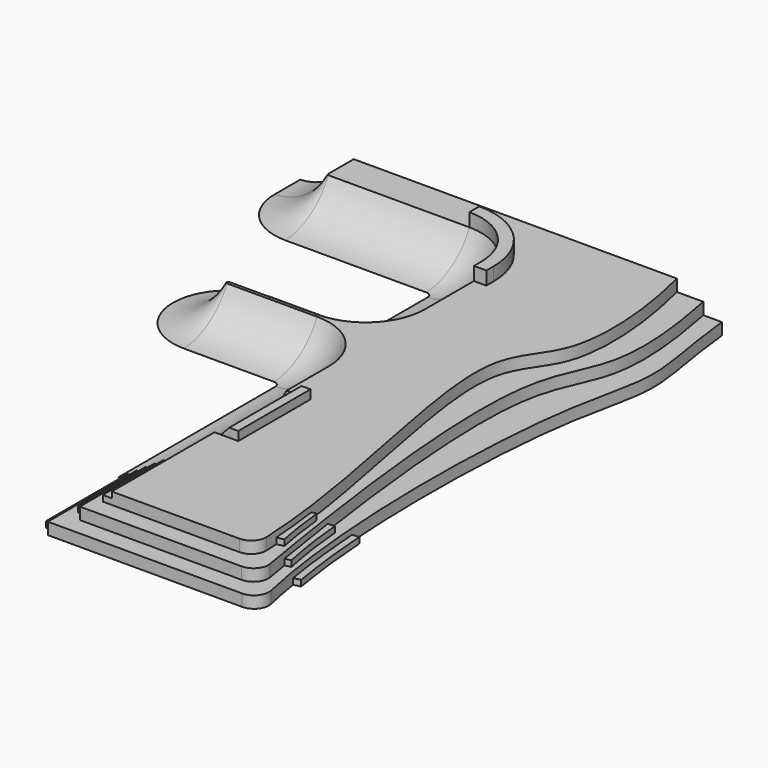
from build123d import *

# Parameters (mm, degrees)
F1_DEPTH  = 1200
F0_W      = 300
F0_H      = 2547.2870769622
F2_DEPTH  = 1000
F3_DEPTH  = 800
F4_DEPTH  = 400
F0_H_2    = 3447.2870769622
F5_DEPTH  = 200
F0_H_3    = 2847.2870769622
F6_DEPTH  = 600
F7_DEPTH  = 200
F8_DEPTH  = 600
F9_DEPTH  = 1000
F16_DEPTH = 1524
F17_DEPTH = 1524
F19_DEPTH = 1200
F21_DEPTH = 450


# Not quite as in the source:
# - a feature names something its author has since deleted; it is built from what else it names


with BuildPart() as f1:
    # F0 (on Top) → F1 (new body)
    with BuildSketch(Plane.XY):
        with BuildLine():
            add(Edge.make_bspline(
                [(8036.4767474961, 10000), (8470.360187732, 8329.6323969196), (8825.7729510838, 4902.0254055318), (6395.2285988216, 3439.3794917817), (8125.3995442021, -2476.6123096312), (8613.2334310908, -6148.2885131691)],
                knots=[0, 0, 0, 0, 0.3059270672, 0.5172086345, 0.9042918919, 0.9042918919, 0.9042918919, 0.9042918919], degree=3))
            Line((8036.4767474961, 10000), (4000, 10000))
            Line((4000, 10000), (4000, -6262.3690662263))
            Line((4000, -6262.3690662263), (4000, -8809.6561431885))
            Line((4000, -8809.6561431885), (8313.2095440952, -8809.6561431885))
            ThreePointArc((8313.2095440952, -8809.6561431885), (8674.6718087547, -8655.1196452075), (8812.6976232832, -8287.0362680974))
            add(Edge.make_bspline(
                [(8787.8384059317, -7848.2893931684), (8797.784205551, -7995.4454937091), (8806.1180126829, -8141.7464710797), (8812.6976232832, -8287.0362680974)],
                knots=[0.9647293852, 0.9647293852, 0.9647293852, 0.9647293852, 0.9806900234, 0.9806900234, 0.9806900234, 0.9806900234], degree=3))
            add(Edge.make_bspline(
                [(8613.2334310908, -6148.2885131691), (8689.4016886612, -6721.5680378242), (8750.1770548915, -7291.0594295347), (8787.8384059317, -7848.2893931684)],
                knots=[0.9042918919, 0.9042918919, 0.9042918919, 0.9042918919, 0.9647293852, 0.9647293852, 0.9647293852, 0.9647293852], degree=3))
        make_face()
    extrude(amount=F1_DEPTH)

    # F0 (on Top) → F2 (join)
    with BuildSketch(Plane.XY):
        with Locations((3850, -7536.0126047074)):
            Rectangle(F0_W, F0_H)
    extrude(amount=F2_DEPTH)

    # F0 (on Top) → F3 (join)
    with BuildSketch(Plane.XY):
        with BuildLine():
            add(Edge.make_bspline(
                [(8931.2620162964, 10000), (9293.0913160754, 8171.5294795271), (9500.0632293716, 5666.7426139981), (7761.7678229589, 3579.4250276228), (8387.3000385547, -2422.1204070051), (8881.4852022515, -5800.6006208613)],
                knots=[0, 0, 0, 0, 0.2826529688, 0.5104916215, 0.8656069765, 0.8656069765, 0.8656069765, 0.8656069765], degree=3))
            Line((8931.2620162964, 10000), (8036.4767474961, 10000))
            add(Edge.make_bspline(
                [(8036.4767474961, 10000), (8470.360187732, 8329.6323969196), (8825.7729510838, 4902.0254055318), (6395.2285988216, 3439.3794917817), (8125.3995442021, -2476.6123096312), (8613.2334310908, -6148.2885131691)],
                knots=[0, 0, 0, 0, 0.3059270672, 0.5172086345, 0.9042918919, 0.9042918919, 0.9042918919, 0.9042918919], degree=3))
            Line((8613.2334310908, -6148.2885131691), (8765.3897849551, -6118.9868246126))
            ThreePointArc((8765.3897849551, -6118.9868246126), (8769.2917139348, -6119.8642958095), (8771.3021241999, -6123.3216439306))
            add(Edge.make_bspline(
                [(8771.3021241999, -6123.3216439306), (8813.4933748329, -6487.7883786699), (8889.3749215397, -7142.4063040065), (8980.0635134111, -7600.1104032829), (9020.3012339996, -7803.1896360599)],
                knots=[0.0027166629, 0.0027166629, 0.0027166629, 0.0027166629, 0.5575142646, 1, 1, 1, 1], degree=3))
            Line((9020.3012339996, -7803.1896360599), (8787.8384059317, -7848.2893931684))
            add(Edge.make_bspline(
                [(8787.8384059317, -7848.2893931684), (8797.784205551, -7995.4454937091), (8806.1180126829, -8141.7464710797), (8812.6976232832, -8287.0362680974)],
                knots=[0.9647293852, 0.9647293852, 0.9647293852, 0.9647293852, 0.9806900234, 0.9806900234, 0.9806900234, 0.9806900234], degree=3))
            ThreePointArc((8812.6976232832, -8287.0362680974), (8674.6718087547, -8655.1196452075), (8313.2095440952, -8809.6561431885))
            Line((8313.2095440952, -8809.6561431885), (4000, -8809.6561431885))
            Line((4000, -8809.6561431885), (3700, -8809.6561431885))
            Line((3700, -8809.6561431885), (3700, -6262.3690662263))
            Line((3700, -6262.3690662263), (3400, -6262.3690662263))
            Line((3400, -6262.3690662263), (3400, -9109.6561431885))
            Line((3400, -9109.6561431885), (3400, -9409.6561431885))
            Line((3400, -9409.6561431885), (8868.0657153652, -9409.6561431885))
            ThreePointArc((8868.0657153652, -9409.6561431885), (9250.0419437511, -9232.2924104432), (9361.0232533911, -8826.0327869808))
            add(Edge.make_bspline(
                [(9232.6634049447, -8057.3231214569), (9275.6513945538, -8319.0025360325), (9318.5440756349, -8575.6191246537), (9361.0232533911, -8826.0327869808)],
                knots=[0.9470475744, 0.9470475744, 0.9470475744, 0.9470475744, 0.9765767788, 0.9765767788, 0.9765767788, 0.9765767788], degree=3))
            add(Edge.make_bspline(
                [(8881.4852022515, -5800.6006208613), (8994.8194600953, -6575.4064543937), (9114.1039092929, -7335.6196946013), (9232.6634049447, -8057.3231214569)],
                knots=[0.8656069765, 0.8656069765, 0.8656069765, 0.8656069765, 0.9470475744, 0.9470475744, 0.9470475744, 0.9470475744], degree=3))
        make_face()
        with Locations((3850, -7536.0126047074)):
            Rectangle(F0_W, F0_H)
    extrude(amount=F3_DEPTH)

    # F0 (on Top) → F4 (join)
    with BuildSketch(Plane.XY):
        with BuildLine():
            add(Edge.make_bspline(
                [(9560.0433349609, 10000), (9738.6629226993, 8251.3060611052), (10297.4382102532, 6478.450699769), (9272.7191558649, 3657.2770747912), (9063.0227701453, -2174.939075243), (9288.8157490666, -5281.5532921831)],
                knots=[0, 0, 0, 0, 0.2568406889, 0.506321619, 0.8252622074, 0.8252622074, 0.8252622074, 0.8252622074], degree=3))
            Line((9560.0433349609, 10000), (8931.2620162964, 10000))
            add(Edge.make_bspline(
                [(8931.2620162964, 10000), (9293.0913160754, 8171.5294795271), (9500.0632293716, 5666.7426139981), (7761.7678229589, 3579.4250276228), (8387.3000385547, -2422.1204070051), (8881.4852022515, -5800.6006208613)],
                knots=[0, 0, 0, 0, 0.2826529688, 0.5104916215, 0.8656069765, 0.8656069765, 0.8656069765, 0.8656069765], degree=3))
            Line((8881.4852022515, -5800.6006208613), (9107.9036665642, -5765.8809567214))
            add(Edge.make_bspline(
                [(9107.9036665642, -5765.8809567214), (9143.5522743599, -6143.655941097), (9214.8742017644, -6899.4677855656), (9360.3479276578, -7645.3727259321), (9433.1099926681, -8018.4544176886)],
                knots=[0, 0, 0, 0, 0.4998267587, 1, 1, 1, 1], degree=3))
            Line((9433.1099926681, -8018.4544176886), (9232.6634049447, -8057.3231214569))
            add(Edge.make_bspline(
                [(9232.6634049447, -8057.3231214569), (9275.6513945538, -8319.0025360325), (9318.5440756349, -8575.6191246537), (9361.0232533911, -8826.0327869808)],
                knots=[0.9470475744, 0.9470475744, 0.9470475744, 0.9470475744, 0.9765767788, 0.9765767788, 0.9765767788, 0.9765767788], degree=3))
            ThreePointArc((9361.0232533911, -8826.0327869808), (9250.0419437511, -9232.2924104432), (8868.0657153652, -9409.6561431885))
            Line((8868.0657153652, -9409.6561431885), (3400, -9409.6561431885))
            Line((3400, -9409.6561431885), (3400, -9109.6561431885))
            Line((3400, -9109.6561431885), (3100, -9109.6561431885))
            Line((3100, -9109.6561431885), (3100, -6262.3690662263))
            Line((3100, -6262.3690662263), (2800, -6262.3690662263))
            Line((2800, -6262.3690662263), (2800, -9709.6561431885))
            Line((2800, -9709.6561431885), (2800, -10009.6561431885))
            Line((2800, -10009.6561431885), (9364.7003943114, -10009.6561431885))
            ThreePointArc((9364.7003943114, -10009.6561431885), (9754.8055196615, -9822.4148220059), (9852.735448729, -9400.928107891))
            add(Edge.make_bspline(
                [(9619.9330184672, -8184.0387894501), (9688.5849810725, -8604.4405106021), (9765.9866472577, -9011.5487180137), (9852.735448729, -9400.928107891)],
                knots=[0.927942243, 0.927942243, 0.927942243, 0.927942243, 0.9748943399, 0.9748943399, 0.9748943399, 0.9748943399], degree=3))
            add(Edge.make_bspline(
                [(9288.8157490666, -5281.5532921831), (9361.507754855, -6281.6996196687), (9469.7973180649, -7264.6578357211), (9619.9330184672, -8184.0387894501)],
                knots=[0.8252622074, 0.8252622074, 0.8252622074, 0.8252622074, 0.927942243, 0.927942243, 0.927942243, 0.927942243], degree=3))
        make_face()
    extrude(amount=F4_DEPTH)

    # F0 (on Top) → F5 (join)
    with BuildSketch(Plane.XY):
        with Locations((2650, -7986.0126047074)):
            Rectangle(F0_W, F0_H_2)
    extrude(amount=F5_DEPTH)

    # F0 (on Top) → F6 (join)
    with BuildSketch(Plane.XY):
        with Locations((3250, -7686.0126047074)):
            Rectangle(F0_W, F0_H_3)
    extrude(amount=F6_DEPTH)

    # F0 (on Top) → F7 (join)
    with BuildSketch(Plane.XY):
        with BuildLine():
            Line((9519.5121765137, -5254.7664642334), (9288.8157490666, -5281.5532921831))
            add(Edge.make_bspline(
                [(9288.8157490666, -5281.5532921831), (9361.507754855, -6281.6996196687), (9469.7973180649, -7264.6578357211), (9619.9330184672, -8184.0387894501)],
                knots=[0.8252622074, 0.8252622074, 0.8252622074, 0.8252622074, 0.927942243, 0.927942243, 0.927942243, 0.927942243], degree=3))
            Line((9619.9330184672, -8184.0387894501), (9853.3172420489, -8129.59868503))
            add(Edge.make_bspline(
                [(9519.5121765137, -5254.7664642334), (9556.921579776, -5743.8481856875), (9631.2627095363, -6715.7665951577), (9779.6168128683, -7660.3444408865), (9853.3172420489, -8129.59868503)],
                knots=[0, 0, 0, 0, 0.5032127354, 1, 1, 1, 1], degree=3))
        make_face()
    extrude(amount=F7_DEPTH)

    # F0 (on Top) → F8 (join)
    with BuildSketch(Plane.XY):
        with BuildLine():
            Line((9107.9036665642, -5765.8809567214), (8881.4852022515, -5800.6006208613))
            add(Edge.make_bspline(
                [(8881.4852022515, -5800.6006208613), (8994.8194600953, -6575.4064543937), (9114.1039092929, -7335.6196946013), (9232.6634049447, -8057.3231214569)],
                knots=[0.8656069765, 0.8656069765, 0.8656069765, 0.8656069765, 0.9470475744, 0.9470475744, 0.9470475744, 0.9470475744], degree=3))
            Line((9232.6634049447, -8057.3231214569), (9433.1099926681, -8018.4544176886))
            add(Edge.make_bspline(
                [(9107.9036665642, -5765.8809567214), (9143.5522743599, -6143.655941097), (9214.8742017644, -6899.4677855656), (9360.3479276578, -7645.3727259321), (9433.1099926681, -8018.4544176886)],
                knots=[0, 0, 0, 0, 0.4998267587, 1, 1, 1, 1], degree=3))
        make_face()
    extrude(amount=F8_DEPTH)

    # F0 (on Top) → F9 (join)
    with BuildSketch(Plane.XY):
        with BuildLine():
            Line((8765.3897849551, -6118.9868246126), (8613.2334310908, -6148.2885131691))
            add(Edge.make_bspline(
                [(8613.2334310908, -6148.2885131691), (8689.4016886612, -6721.5680378242), (8750.1770548915, -7291.0594295347), (8787.8384059317, -7848.2893931684)],
                knots=[0.9042918919, 0.9042918919, 0.9042918919, 0.9042918919, 0.9647293852, 0.9647293852, 0.9647293852, 0.9647293852], degree=3))
            Line((8787.8384059317, -7848.2893931684), (9020.3012339996, -7803.1896360599))
            add(Edge.make_bspline(
                [(8771.3021241999, -6123.3216439306), (8813.4933748329, -6487.7883786699), (8889.3749215397, -7142.4063040065), (8980.0635134111, -7600.1104032829), (9020.3012339996, -7803.1896360599)],
                knots=[0.0027166629, 0.0027166629, 0.0027166629, 0.0027166629, 0.5575142646, 1, 1, 1, 1], degree=3))
            ThreePointArc((8771.3021241999, -6123.3216439306), (8769.2917139348, -6119.8642958095), (8765.3897849551, -6118.9868246126))
        make_face()
    extrude(amount=F9_DEPTH)

    # F12: sweep along a path in F0
    with BuildLine(Plane.XY) as f12_path:
        Line((2240.3030395508, -6262.3690662263), (2240.3030395508, 358.4062457085))
        ThreePointArc((2240.3030395508, 358.4062457085), (2167.0797348474, 535.1829410051), (1990.3030395508, 608.4062457085))
        Line((1990.3030395508, 608.4062457085), (-1051.7582893372, 608.4062457085))
        ThreePointArc((-1051.7582893372, 608.4062457085), (-2863.7582893372, 2420.4062457085), (-1051.7582893372, 4232.4062457085))
        Line((-1051.7582893372, 4232.4062457085), (1938, 4232.4062457085))
        ThreePointArc((1938, 4232.4062457085), (2114.7766952966, 4305.6295504118), (2188, 4482.4062457085))
        Line((2188, 4482.4062457085), (2188, 6856.2393188477))
        ThreePointArc((2188, 6856.2393188477), (2114.7766952966, 7033.0160141443), (1938, 7106.2393188477))
        Line((1938, 7106.2393188477), (-2824.0236428859, 7106.2393188477))
        ThreePointArc((-2824.0236428859, 7106.2393188477), (-4105.3011303959, 7636.9618313376), (-4636.0236428859, 8918.2393188477))
        Line((-4636.0236428859, 8918.2393188477), (-4636.0236428859, 10000))
    # F11 (on line) → F12 (sweep)
    with BuildSketch(Plane(origin=(0, -6262.3690662263, 0), x_dir=(-1, 0, 0), z_dir=(0, 1, 0))):
        with BuildLine():
            ThreePointArc((-2187.540769577, 0), (-3258.099588071, 351.8000155689), (-4000, 1200))
            Line((-4000, 1200), (-4000, 1000))
            Line((-4000, 1000), (-4000, 0))
            Line((-4000, 0), (-2187.540769577, 0))
        make_face()
    sweep(path=f12_path.line)

    # F15 (on face) → F16 (join, symmetric)
    with BuildSketch(Plane(origin=(0, -2951.9814102589, 0), x_dir=(-1, 0, 0), z_dir=(0, 1, 0))):
        Polygon((-4225.5687713623, 1200), (-4500.6198883057, 1500), (-4805.4198883057, 1500), (-4805.4198883057, 1200), align=None)
    extrude(amount=F16_DEPTH, both=True)

    # F15 (on face) → F17 (cut, symmetric)
    with BuildSketch(Plane(origin=(0, -2951.9814102589, 0), x_dir=(-1, 0, 0), z_dir=(0, 1, 0))):
        Polygon((-3236.7072105408, 1854.6521663666), (-4225.5687713623, 1200), (-3485.6019020081, 525.5545377731), (-1603.2665967941, 735.3942990303), align=None)
    extrude(amount=F17_DEPTH, both=True, mode=Mode.SUBTRACT)

    # F18 (on face) → F19 (join)
    with BuildSketch(Plane(origin=(0, 0, 0), x_dir=(1, 0, 0), z_dir=(0, 0, -1))):
        with BuildLine():
            Line((-2876.3266824367, -10000), (4000, -10000))
            Line((4000, -10000), (4000, -358.4062457085))
            ThreePointArc((4000, -358.4062457085), (3411.3733884144, -1779.4765945721), (1990.3030395508, -2368.1032061577))
            Line((1990.3030395508, -2368.1032061577), (-1051.7582893372, -2368.1032061577))
            ThreePointArc((-1051.7582893372, -2368.1032061577), (-1104.0613288879, -2420.4062457085), (-1051.7582893372, -2472.7092852592))
            Line((-1051.7582893372, -2472.7092852592), (1938, -2472.7092852592))
            ThreePointArc((1938, -2472.7092852592), (3359.0703488636, -3061.3358968448), (3947.6969604492, -4482.4062457084))
            Line((3947.6969604492, -4482.4062457084), (3947.6969604492, -6856.2393188476))
            ThreePointArc((3947.6969604492, -6856.2393188476), (3359.0703488637, -8277.3096677112), (1938.0000000002, -8865.9362792969))
            Line((1938.0000000002, -8865.9362792969), (-2824.0236428857, -8865.9362792969))
            ThreePointArc((-2824.0236428857, -8865.9362792969), (-2861.0074768288, -8881.2554849045), (-2876.3266824367, -8918.2393188475))
            Line((-2876.3266824367, -8918.2393188475), (-2876.3266824367, -9999.9999999998))
        make_face()
    extrude(amount=-F19_DEPTH)

    # F20 (on face) → F21 (join)
    with BuildSketch(Plane.XY.offset(1200)):
        with BuildLine():
            ThreePointArc((1938, 8865.9362792969), (3359.0703488636, 8277.3096677113), (3947.6969604492, 6856.2393188477))
            Line((3947.6969604492, 6856.2393188477), (3947.6969604492, 6544.5799827576))
            Line((3947.6969604492, 6544.5799827576), (4367.6966701962, 6544.5799827576))
            Line((4367.6966701962, 6544.5799827576), (4367.6966701962, 6856.2393188477))
            ThreePointArc((4367.6966701962, 6856.2393188477), (3656.0549917221, 8574.2943105698), (1938, 9285.9359890439))
            Line((1938, 9285.9359890439), (1938, 8865.9362792969))
        make_face()
    extrude(amount=F21_DEPTH)


solid = f1.part
